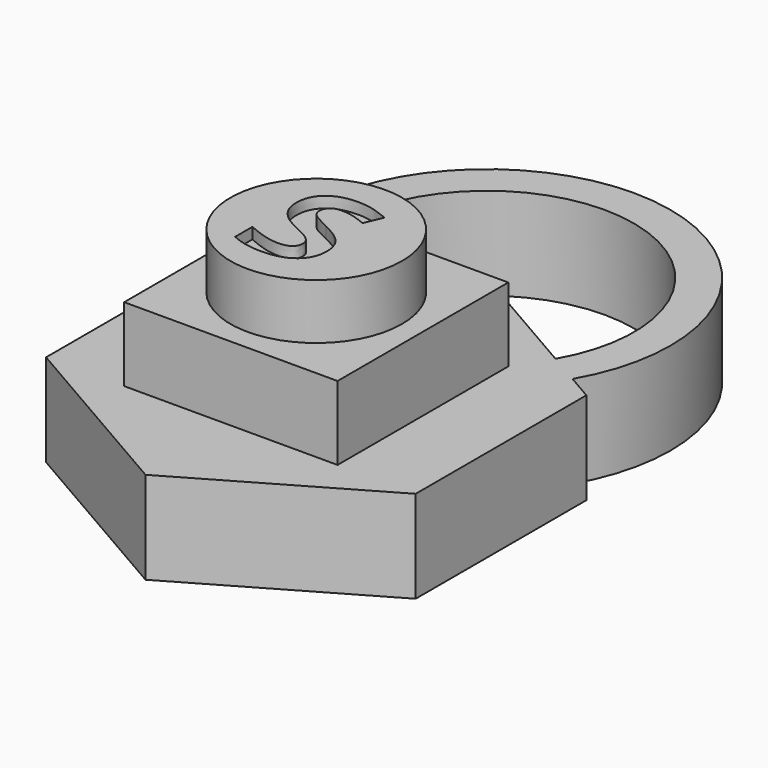
from build123d import *

# Parameters (mm, degrees)
F1_DEPTH     = 6.35
F2_W         = 14.6646968374
F2_H         = 14.6646968374
F3_DEPTH     = 5.08
F4_R         = 5.8973186229
F5_DEPTH     = 3.81
F6_TEXT_SIZE = 10.535631898
F7_DEPTH     = 0.762
F8_R         = 12.6245872647
F8_R_2       = 10.1107162358
F9_DEPTH     = 6.35


# Not quite as in the source:
# - Text() gives the source's letters only with a copy of the font that has no kerning and outlines rounded to 1/6400 em; it was checked with that copy


with BuildPart() as f1:
    # F0 (on Top) → F1 (new body)
    with BuildSketch(Plane.XY):
        Polygon((12.7, -7.3323484187), (12.7, 7.3323484187), (0, 14.6646968374), (-12.7, 7.3323484187), (-12.7, -7.3323484187), (0, -14.6646968374), align=None)
    extrude(amount=F1_DEPTH)

    # F2 (on face) → F3 (join)
    with BuildSketch(Plane.XY.offset(6.35)):
        Rectangle(F2_W, F2_H)
    extrude(amount=F3_DEPTH)

    # F4 (on face) → F5 (join)
    with BuildSketch(Plane.XY.offset(11.43)):
        Circle(F4_R)
    extrude(amount=F5_DEPTH)

    # F6 (on face) → F7 (cut)
    with BuildSketch(Plane.XY.offset(15.24)):
        with Locations((-3.3416023944, -3.7417525891)):
            Text('S', F6_TEXT_SIZE, font='Open Sans', font_style=FontStyle.BOLD, text_align=(TextAlign.LEFT, TextAlign.BOTTOM))
    extrude(amount=-F7_DEPTH, mode=Mode.SUBTRACT)

    # F8 (on face) → F9 (join, through all)
    with BuildSketch(Plane.XY.offset(6.35)):
        with Locations((0, 14.6646968374)):
            Circle(F8_R)
        with Locations((0, 14.6646968374)):
            Circle(F8_R_2, mode=Mode.SUBTRACT)
    extrude(amount=-F9_DEPTH)


solid = f1.part
